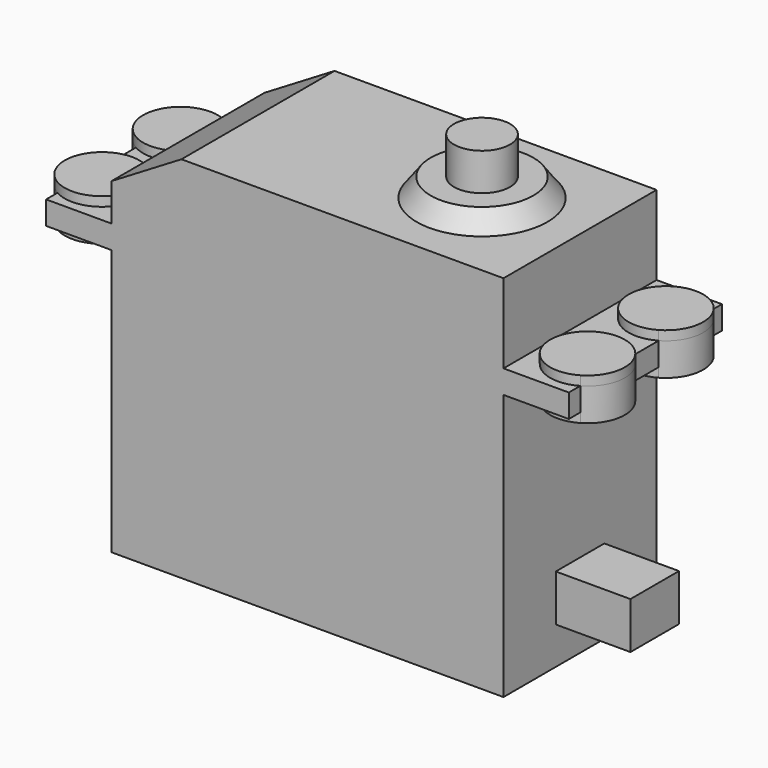
from build123d import *

# Parameters (mm, degrees)
F0_W          = 20.5
F0_H          = 42
F1_DEPTH      = 39.5
F2_START      = 8.5
F2_DEPTH      = 2.5
F5_W          = 6.5
F5_H          = 5
F6_DEPTH      = 8
F7_SIZE2      = 4.5
F7_SIZE       = 7.5
F8_R          = 4
F9_DEPTH      = 1
F9_DEPTH_BACK = 3.5
F10_ANGLE     = 180
F12_ANGLE     = -90


# Not quite as in the source:
# - a feature names something its author has since deleted; it is built from what else it names


with BuildPart() as f1:
    # F0 (on Top) → F1 (new body)
    with BuildSketch(Plane.XY):
        with Locations((0, -10.5)):
            Rectangle(F0_W, F0_H)
    extrude(amount=F1_DEPTH)

    # F0 (on Top) → F2 (join)
    with BuildSketch(Plane.XY.offset(F2_START)):
        with BuildLine():
            Line((-10.25, 10.5), (10.25, 10.5))
            Line((10.25, 10.5), (10.25, 17.5))
            Line((10.25, 17.5), (6.2807764064, 17.5))
            ThreePointArc((6.2807764064, 17.5), (5.25, 13.25), (4.2192235936, 17.5))
            Line((4.2192235936, 17.5), (-4.2192235936, 17.5))
            ThreePointArc((-4.2192235936, 17.5), (-5.25, 13.25), (-6.2807764064, 17.5))
            Line((-6.2807764064, 17.5), (-10.25, 17.5))
            Line((-10.25, 17.5), (-10.25, 10.5))
        make_face()
        with BuildLine():
            Line((10.25, -38.5), (10.25, -31.5))
            Line((10.25, -31.5), (-10.25, -31.5))
            Line((-10.25, -31.5), (-10.25, -38.5))
            Line((-10.25, -38.5), (-6.2807764064, -38.5))
            ThreePointArc((-6.2807764064, -38.5), (-5.25, -34.25), (-4.2192235936, -38.5))
            Line((-4.2192235936, -38.5), (4.2192235936, -38.5))
            ThreePointArc((4.2192235936, -38.5), (5.25, -34.25), (6.2807764064, -38.5))
            Line((6.2807764064, -38.5), (10.25, -38.5))
        make_face()
    extrude(amount=F2_DEPTH)

    # F3 (on Right) → F4 (revolve)
    with BuildSketch(Plane.YZ):
        Polygon((5.5, -2), (7, 0), (0, 0), (0, -6), (3, -6), (3, -2), align=None)
    revolve(axis=Axis((0, 0, -3), (0, 0, 1)))

    # F5 (on face) → F6 (join)
    with BuildSketch(Plane(origin=(0, 10.5, 0), x_dir=(-1, 0, 0), z_dir=(0, 1, 0))):
        with Locations((0, 33)):
            Rectangle(F5_W, F5_H)
    extrude(amount=F6_DEPTH)

    # F7
    f7_edges = [f1.edges().sort_by_distance(p)[0] for p in [
        (0, -31.5, 0),
    ]]
    f7_side = f1.faces().sort_by_distance((0, -12.786008, 0))[0]
    chamfer(f7_edges, length=F7_SIZE, length2=F7_SIZE2, reference=f7_side)

    # F8 (on face) → F9 (join, two sides)
    with BuildSketch(Plane(origin=(0, 0, 8.5), x_dir=(1, 0, 0), z_dir=(0, 0, -1))) as f9_sk:
        with Locations((-5.25, 36.5)):
            Circle(F8_R)
        with Locations((5.25, 36.5)):
            Circle(F8_R)
        with BuildLine():
            Line((4.2192235936, -17.5), (1.7858983849, -17.5))
            ThreePointArc((1.7858983849, -17.5), (5.25, -19.5), (8.7141016151, -17.5))
            Line((8.7141016151, -17.5), (6.2807764064, -17.5))
            ThreePointArc((6.2807764064, -17.5), (5.25, -13.25), (4.2192235936, -17.5))
        make_face()
        with BuildLine():
            Line((-8.7141016151, -17.5), (-6.2807764064, -17.5))
            ThreePointArc((-6.2807764064, -17.5), (-5.25, -13.25), (-4.2192235936, -17.5))
            Line((-4.2192235936, -17.5), (-1.7858983849, -17.5))
            ThreePointArc((-1.7858983849, -17.5), (-1.3862966948, -16.5352761804), (-1.25, -15.5))
            ThreePointArc((-1.25, -15.5), (-6.2852761804, -11.6362966948), (-8.7141016151, -17.5))
        make_face()
        with BuildLine():
            ThreePointArc((-4.2192235936, -17.5), (-5.25, -13.25), (-6.2807764064, -17.5))
            Line((-6.2807764064, -17.5), (-8.7141016151, -17.5))
            ThreePointArc((-8.7141016151, -17.5), (-5.25, -19.5), (-1.7858983849, -17.5))
            Line((-1.7858983849, -17.5), (-4.2192235936, -17.5))
        make_face()
        with BuildLine():
            ThreePointArc((9.25, -15.5), (4.2147238196, -11.6362966948), (1.7858983849, -17.5))
            Line((1.7858983849, -17.5), (4.2192235936, -17.5))
            ThreePointArc((4.2192235936, -17.5), (5.25, -13.25), (6.2807764064, -17.5))
            Line((6.2807764064, -17.5), (8.7141016151, -17.5))
            ThreePointArc((8.7141016151, -17.5), (9.1137033052, -16.5352761804), (9.25, -15.5))
        make_face()
    extrude(amount=F9_DEPTH)
    extrude(f9_sk.sketch, amount=-F9_DEPTH_BACK)


with BuildPart() as f1_1:
    # F10: moved
    add(f1.part.rotate(Axis((0, 5.25, 0), (0, 1, 0)), F10_ANGLE))


with BuildPart() as f1_2:
    # F11: moved
    add(f1_1.part.moved(Location((0, 0, -6))))


with BuildPart() as f1_3:
    # F12: moved
    add(f1_2.part.rotate(Axis((0, 0, -3), (0, 0, 1)), F12_ANGLE))


solid = f1_3.part
